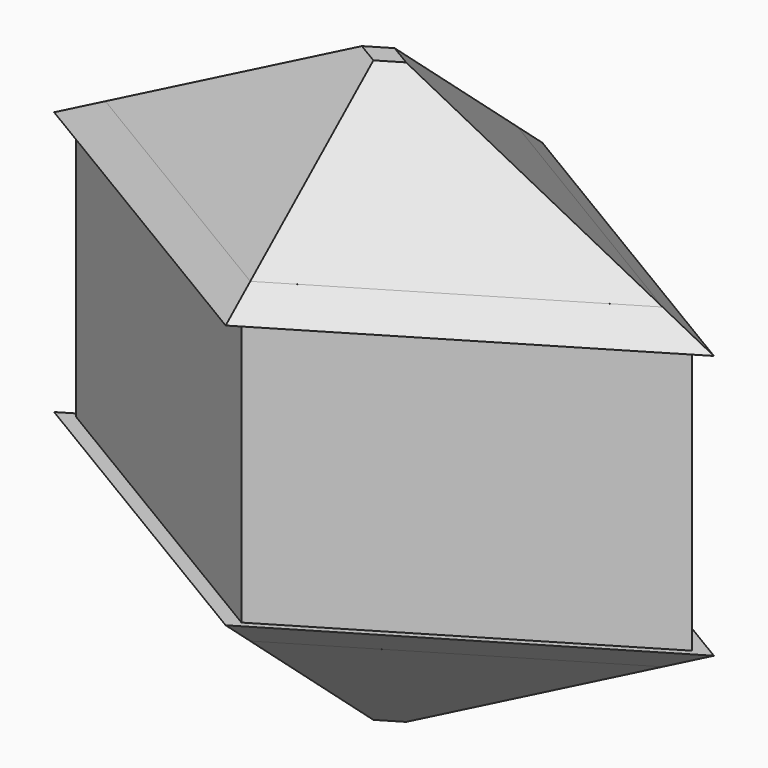
from build123d import *

# Parameters (mm, degrees)
F1_DEPTH  = 4.318
F2_DEPTH  = 1.778
F3_SIZE   = 0.508
F4_SIZE   = 0.508
F5_SIZE   = 0.508
F6_DEPTH  = 2.54
F7_DEPTH  = 2.54
F8_SIZE   = 2.53999
F9_SIZE   = 2.53999
F11_DEPTH = 0.254
F12_DEPTH = 0.254


# Not quite as in the source:
# - a fillet or chamfer is up to 0.001 mm smaller than in the source, because OpenCascade refuses the exact size
# - a feature names something its author has since deleted; it is built from what else it names


with BuildPart() as f1:
    # F0 (on Top) → F1 (new body)
    with BuildSketch(Plane.XY):
        Polygon((-6.35, 0), (0, 0), (0, 3.81), align=None)
        Polygon((0, 3.81), (0, 0), (6.35, 0), align=None)
        Polygon((6.35, 0), (0, 0), (0, -3.81), align=None)
        Polygon((0, -3.81), (0, 0), (-6.35, 0), align=None)
    extrude(amount=F1_DEPTH)

    # F5
    f5_edges = [f1.edges().sort_by_distance(p)[0] for p in [
        (-3.175, -1.905, 4.318),
        (3.175, -1.905, 4.318),
        (3.175, 1.905, 4.318),
        (-3.175, 1.905, 4.318),
    ]]
    chamfer(f5_edges, length=F5_SIZE)

    # F7 (add): a face of the model
    f7_faces = [f1.faces().sort_by_distance(p)[0] for p in [
        (0, 0, 4.318),
    ]]
    extrude(f7_faces, amount=F7_DEPTH)

    # F8 (size 2.54 in the source; OpenCascade refuses exactly that, so slightly less here)
    f8_edges = [f1.edges().sort_by_distance(p)[0] for p in [
        (-2.681313, -1.608788, 6.858),
        (-2.681313, 1.608788, 6.858),
        (2.681313, -1.608788, 6.858),
        (2.681313, 1.608788, 6.858),
    ]]
    chamfer(f8_edges, length=F8_SIZE)


with BuildPart() as f2:
    # F0 (on Top) → F2 (new body)
    with BuildSketch(Plane.XY):
        Polygon((6.35, 0), (0, 0), (0, -3.81), align=None)
        Polygon((0, -3.81), (0, 0), (-6.35, 0), align=None)
        Polygon((0, 3.81), (0, 0), (6.35, 0), align=None)
        Polygon((-6.35, 0), (0, 0), (0, 3.81), align=None)
    extrude(amount=-F2_DEPTH)

    # F3
    f3_edges = [f2.edges().sort_by_distance(p)[0] for p in [
        (3.175, 1.905, -1.778),
        (3.175, -1.905, -1.778),
    ]]
    chamfer(f3_edges, length=F3_SIZE)

    # F4
    f4_edges = [f2.edges().sort_by_distance(p)[0] for p in [
        (-3.421844, 1.756894, -1.778),
        (-3.421844, -1.756894, -1.778),
    ]]
    chamfer(f4_edges, length=F4_SIZE)

    # F6 (add): a face of the model
    f6_faces = [f2.faces().sort_by_distance(p)[0] for p in [
        (0, 0, -1.778),
    ]]
    extrude(f6_faces, amount=F6_DEPTH)

    # F9 (size 2.54 in the source; OpenCascade refuses exactly that, so slightly less here)
    f9_edges = [f2.edges().sort_by_distance(p)[0] for p in [
        (2.681313, 1.608788, -4.318),
        (-2.681313, 1.608788, -4.318),
        (2.681313, -1.608788, -4.318),
        (-2.681313, -1.608788, -4.318),
    ]]
    chamfer(f9_edges, length=F9_SIZE)

    # F10: union F1
    add(f1.part)

    # F11 (cut): faces of the model
    f11_faces = [f2.faces().sort_by_distance(p)[0] for p in [
        (3.175, 1.905, 1.27),
        (-3.175, 1.905, 1.27),
        (-3.175, -1.905, 1.27),
        (3.175, -1.905, 1.27),
    ]]
    extrude(f11_faces, amount=-F11_DEPTH, dir=(0.5144957554, 0.8574929257, 0), mode=Mode.SUBTRACT)

    # F12 (cut): faces of the model
    f12_faces = [f2.faces().sort_by_distance(p)[0] for p in [
        (-3.1169191458, -1.9398485125, 1.27),
        (3.0515781849, -1.9790530891, 1.27),
    ]]
    extrude(f12_faces, amount=-F12_DEPTH, dir=(-0.5144957554, -0.8574929257, 0), mode=Mode.SUBTRACT)


solid = f2.part
